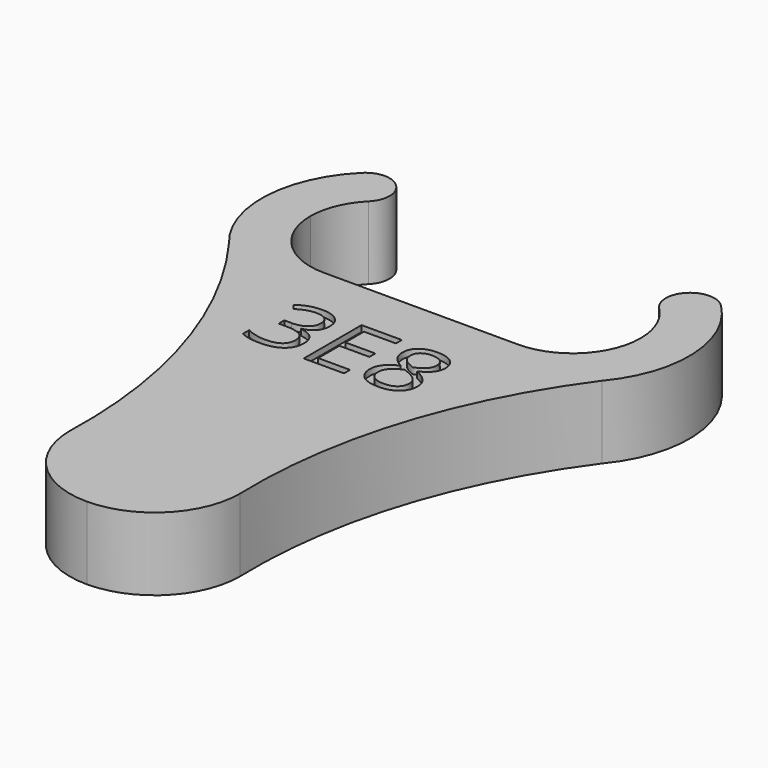
from build123d import *

# Parameters (mm, degrees)
F2_DEPTH     = 6
F3_TEXT_SIZE = 8.3333333333
F4_DEPTH     = 0.5


# Not quite as in the source:
# - Text() gives the source's letters only with a copy of the font that has no kerning and outlines rounded to 1/6400 em; it was checked with that copy


with BuildPart() as f2:
    # F1 (on Top) → F2 (new body)
    with BuildSketch(Plane.XY):
        with BuildLine():
            ThreePointArc((-8, -5.6), (-11.9597979746, -3.9597979746), (-13.6, 0))
            ThreePointArc((-13.6, 0), (-13.1737253821, 2.1430272212), (-11.9597979746, 3.9597979746))
            ThreePointArc((-11.9597979746, 3.9597979746), (-11.9597979746, 6.7882250994), (-14.7882250994, 6.7882250994))
            ThreePointArc((-14.7882250994, 6.7882250994), (-17.5908629272, 0.4187461187), (-15.3540266539, -6.170761053))
            ThreePointArc((-15.3540266539, -6.170761053), (-8.9236154136, -18.8837226723), (-7, -33))
            ThreePointArc((-7, -33), (-4.9497474683, -37.9497474683), (0, -40))
            ThreePointArc((0, -40), (4.9497474683, -37.9497474683), (7, -33))
            ThreePointArc((7, -33), (8.9236154136, -18.8837226723), (15.3540266539, -6.170761053))
            ThreePointArc((15.3540266539, -6.170761053), (17.5908629272, 0.4187461187), (14.7882250994, 6.7882250994))
            ThreePointArc((14.7882250994, 6.7882250994), (11.9597979746, 6.7882250994), (11.9597979746, 3.9597979746))
            ThreePointArc((11.9597979746, 3.9597979746), (13.1737253821, 2.1430272212), (13.6, 0))
            ThreePointArc((13.6, 0), (11.9597979746, -3.9597979746), (8, -5.6))
            Line((8, -5.6), (0, -5.6))
            Line((0, -5.6), (-8, -5.6))
        make_face()
    extrude(amount=F2_DEPTH)

    # F3 (on face) → F4 (cut)
    with BuildSketch(Plane.XY.offset(6)):
        with Locations((-7.1360677083, -15.7292176739)):
            Text('3E8', F3_TEXT_SIZE, font='Open Sans', text_align=(TextAlign.LEFT, TextAlign.BOTTOM))
    extrude(amount=-F4_DEPTH, mode=Mode.SUBTRACT)


solid = f2.part
